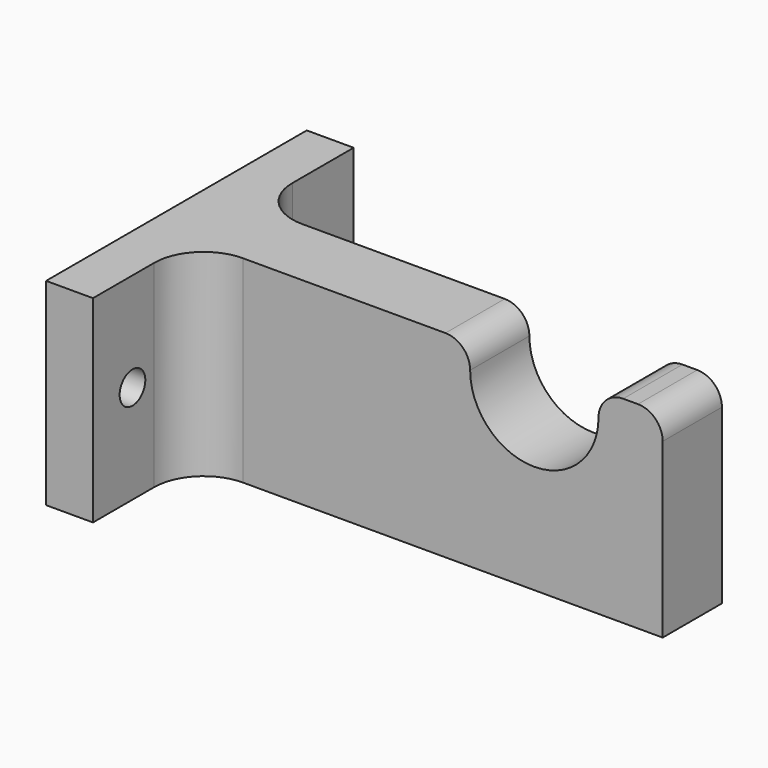
from build123d import *

# Parameters (mm, degrees)
F1_DEPTH = 40
F2_R     = 3.25
F3_DEPTH = 104.501
F5_DEPTH = 40.501
F6_R     = 10
F7_R     = 4.99999
F8_R     = 5


# Not quite as in the source:
# - a fillet or chamfer is up to 0.001 mm smaller than in the source, because OpenCascade refuses the exact size


with BuildPart() as f1:
    # F0 (on Top) → F1 (new body)
    with BuildSketch(Plane.XY):
        Polygon((0, 66), (0, 0), (9.5, 0), (9.5, 25.5), (104.5, 25.5), (104.5, 40.5), (9.5, 40.5), (9.5, 66), align=None)
    extrude(amount=F1_DEPTH)

    # F2 (on face) → F3 (cut, through all)
    with BuildSketch(Plane(origin=(0, 0, 0), x_dir=(0, -1, 0), z_dir=(-1, 0, 0))):
        with Locations((-56, 20)):
            Circle(F2_R)
        with Locations((-10, 20)):
            Circle(F2_R)
    extrude(amount=-F3_DEPTH, mode=Mode.SUBTRACT)

    # F4 (on face) → F5 (cut, through all)
    with BuildSketch(Plane.XZ.offset(-25.5)):
        with BuildLine():
            Line((65.5, 35), (91.5, 35))
            ThreePointArc((91.5, 35), (78.5, 48), (65.5, 35))
        make_face()
        with BuildLine():
            ThreePointArc((65.5, 35), (78.5, 22), (91.5, 35))
            Line((91.5, 35), (65.5, 35))
        make_face()
        with BuildLine():
            ThreePointArc((65.5, 35), (78.5, 48), (91.5, 35))
            Line((91.5, 35), (91.5, 50.4635125536))
            Line((91.5, 50.4635125536), (65.5, 50.4635125536))
            Line((65.5, 50.4635125536), (65.5, 35))
        make_face()
    extrude(amount=-F5_DEPTH, mode=Mode.SUBTRACT)

    # F6
    f6_edges = [f1.edges().sort_by_distance(p)[0] for p in [
        (9.5, 25.5, 20),
        (9.5, 40.5, 20),
    ]]
    fillet(f6_edges, radius=F6_R)

    # F7 (radius 5 in the source; OpenCascade refuses exactly that, so slightly less here)
    f7_edges = [f1.edges().sort_by_distance(p)[0] for p in [
        (65.5, 33, 40),
        (91.5, 33, 40),
    ]]
    fillet(f7_edges, radius=F7_R)

    # F8
    f8_edges = [f1.edges().sort_by_distance(p)[0] for p in [
        (104.5, 33, 40),
    ]]
    fillet(f8_edges, radius=F8_R)


solid = f1.part
